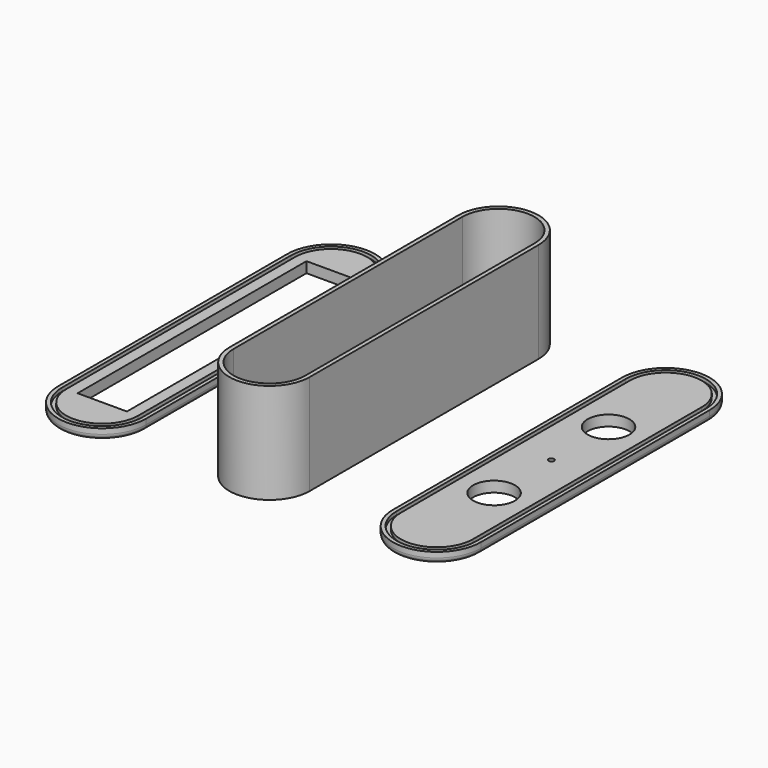
from build123d import *

# Parameters (mm, degrees)
F4_DEPTH  = 12.7
F3_W      = 59
F3_H      = 342.0000019477
F5_DEPTH  = 8.4666666667
F6_D      = 50
F7_D      = 6.5
F9_DEPTH  = 12.7
F10_DEPTH = 8.4666666667
F12_DEPTH = 120
F13_DEPTH = 4.5
F14_D     = 3.5
F15_R     = 6.35
F15_2_R   = 6.35


# Not quite as in the source:
# - a feature names something its author has since deleted; it is built from what else it names


with BuildPart() as f4:
    # F3 (on Top) → F4 (new body)
    with BuildSketch(Plane.XY):
        with BuildLine():
            Line((105, -171), (105, 0))
            Line((105, 0), (105, 171))
            ThreePointArc((105, 171), (52.5, 223.5), (0, 171))
            Line((0, 171), (0, 0))
            Line((0, 0), (0, -171))
            ThreePointArc((0, -171), (52.5, -223.5), (105, -171))
        make_face()
        with BuildLine():
            Line((100.5, 171), (100.5, 0))
            Line((100.5, 0), (100.5, -171))
            ThreePointArc((100.5, -171), (52.5, -219), (4.5, -171))
            Line((4.5, -171), (4.5, 0))
            Line((4.5, 0), (4.5, 171))
            ThreePointArc((4.5, 171), (52.5, 219), (100.5, 171))
        make_face(mode=Mode.SUBTRACT)
    extrude(amount=F4_DEPTH)



with BuildPart() as f4b:
    # F3 (on Top) → F4, piece 2 (new body)
    with BuildSketch(Plane.XY):
        with BuildLine():
            Line((9.5, 171.0000009738), (9.5, 0))
            Line((9.5, 0), (9.5, -171.0000009738))
            ThreePointArc((9.5, -171.0000009738), (52.5, -214), (95.5, -171.0000009738))
            Line((95.5, -171.0000009738), (95.5, 0))
            Line((95.5, 0), (95.5, 171.0000009738))
            ThreePointArc((95.5, 171.0000009738), (52.5, 214), (9.5, 171.0000009738))
        make_face()
        with Locations((52.5, 0)):
            Rectangle(F3_W, F3_H, mode=Mode.SUBTRACT)
        with Locations((52.5, 0)):
            Rectangle(F3_W, F3_H)
    extrude(amount=F4_DEPTH)


with BuildPart() as f4_1:
    add(f4.part)

    add(f4b.part)  # F5 merges F4b
    # F3 (on Top) → F5 (join)
    with BuildSketch(Plane.XY):
        with BuildLine():
            Line((105, -171), (105, 0))
            Line((105, 0), (105, 171))
            ThreePointArc((105, 171), (52.5, 223.5), (0, 171))
            Line((0, 171), (0, 0))
            Line((0, 0), (0, -171))
            ThreePointArc((0, -171), (52.5, -223.5), (105, -171))
        make_face()
        with BuildLine():
            Line((100.5, 171), (100.5, 0))
            Line((100.5, 0), (100.5, -171))
            ThreePointArc((100.5, -171), (52.5, -219), (4.5, -171))
            Line((4.5, -171), (4.5, 0))
            Line((4.5, 0), (4.5, 171))
            ThreePointArc((4.5, 171), (52.5, 219), (100.5, 171))
        make_face(mode=Mode.SUBTRACT)
        with BuildLine():
            Line((100.5, -171), (100.5, 0))
            Line((100.5, 0), (100.5, 171))
            ThreePointArc((100.5, 171), (52.5, 219), (4.5, 171))
            Line((4.5, 171), (4.5, 0))
            Line((4.5, 0), (4.5, -171))
            ThreePointArc((4.5, -171), (52.5, -219), (100.5, -171))
        make_face()
        with BuildLine():
            Line((9.5, -171.0000009738), (9.5, 0))
            Line((9.5, 0), (9.5, 171.0000009738))
            ThreePointArc((9.5, 171.0000009738), (52.5, 214), (95.5, 171.0000009738))
            Line((95.5, 171.0000009738), (95.5, 0))
            Line((95.5, 0), (95.5, -171.0000009738))
            ThreePointArc((95.5, -171.0000009738), (52.5, -214), (9.5, -171.0000009738))
        make_face(mode=Mode.SUBTRACT)
        with BuildLine():
            Line((9.5, 171.0000009738), (9.5, 0))
            Line((9.5, 0), (9.5, -171.0000009738))
            ThreePointArc((9.5, -171.0000009738), (52.5, -214), (95.5, -171.0000009738))
            Line((95.5, -171.0000009738), (95.5, 0))
            Line((95.5, 0), (95.5, 171.0000009738))
            ThreePointArc((95.5, 171.0000009738), (52.5, 214), (9.5, 171.0000009738))
        make_face()
        with Locations((52.5, 0)):
            Rectangle(F3_W, F3_H, mode=Mode.SUBTRACT)
    extrude(amount=F5_DEPTH)

    # F6 (through all)
    with Locations(Plane(origin=(0, 0, 0), x_dir=(1, 0, 0), z_dir=(0, 0, -1))):
        with Locations((52.5, 85.5), (52.5, -85.5)):
            Hole(F6_D / 2)

    # F7 (through all)
    with Locations(Plane(origin=(0, 0, 0), x_dir=(1, 0, 0), z_dir=(0, 0, -1))):
        with Locations((52.5, 0)):
            Hole(F7_D / 2)


with BuildPart() as f4_2:
    # F8: moved
    add(f4_1.part.moved(Location((200, 0, 0))))

    # F15
    f15_edges = [f4_2.edges().sort_by_distance(p)[0] for p in [
        (200, 0, 0),
    ]]
    fillet(f15_edges, radius=F15_R)


with BuildPart() as f9:
    # F3 (on Top) → F9 (new body)
    with BuildSketch(Plane.XY):
        with BuildLine():
            Line((105, -171), (105, 0))
            Line((105, 0), (105, 171))
            ThreePointArc((105, 171), (52.5, 223.5), (0, 171))
            Line((0, 171), (0, 0))
            Line((0, 0), (0, -171))
            ThreePointArc((0, -171), (52.5, -223.5), (105, -171))
        make_face()
        with BuildLine():
            Line((100.5, 171), (100.5, 0))
            Line((100.5, 0), (100.5, -171))
            ThreePointArc((100.5, -171), (52.5, -219), (4.5, -171))
            Line((4.5, -171), (4.5, 0))
            Line((4.5, 0), (4.5, 171))
            ThreePointArc((4.5, 171), (52.5, 219), (100.5, 171))
        make_face(mode=Mode.SUBTRACT)
    extrude(amount=F9_DEPTH)



with BuildPart() as f9b:
    # F3 (on Top) → F9, piece 2 (new body)
    with BuildSketch(Plane.XY):
        with BuildLine():
            Line((9.5, 171.0000009738), (9.5, 0))
            Line((9.5, 0), (9.5, -171.0000009738))
            ThreePointArc((9.5, -171.0000009738), (52.5, -214), (95.5, -171.0000009738))
            Line((95.5, -171.0000009738), (95.5, 0))
            Line((95.5, 0), (95.5, 171.0000009738))
            ThreePointArc((95.5, 171.0000009738), (52.5, 214), (9.5, 171.0000009738))
        make_face()
        with Locations((52.5, 0)):
            Rectangle(F3_W, F3_H, mode=Mode.SUBTRACT)
    extrude(amount=F9_DEPTH)


with BuildPart() as f9_1:
    add(f9.part)

    add(f9b.part)  # F10 merges F9b
    # F3 (on Top) → F10 (join)
    with BuildSketch(Plane.XY):
        with BuildLine():
            Line((100.5, -171), (100.5, 0))
            Line((100.5, 0), (100.5, 171))
            ThreePointArc((100.5, 171), (52.5, 219), (4.5, 171))
            Line((4.5, 171), (4.5, 0))
            Line((4.5, 0), (4.5, -171))
            ThreePointArc((4.5, -171), (52.5, -219), (100.5, -171))
        make_face()
        with BuildLine():
            Line((9.5, -171.0000009738), (9.5, 0))
            Line((9.5, 0), (9.5, 171.0000009738))
            ThreePointArc((9.5, 171.0000009738), (52.5, 214), (95.5, 171.0000009738))
            Line((95.5, 171.0000009738), (95.5, 0))
            Line((95.5, 0), (95.5, -171.0000009738))
            ThreePointArc((95.5, -171.0000009738), (52.5, -214), (9.5, -171.0000009738))
        make_face(mode=Mode.SUBTRACT)
    extrude(amount=F10_DEPTH)


with BuildPart() as f9_2:
    # F11: moved
    add(f9_1.part.moved(Location((-200, 0, 0))))

    # F15#2
    f15_2_edges = [f9_2.edges().sort_by_distance(p)[0] for p in [
        (-95, 0, 0),
    ]]
    fillet(f15_2_edges, radius=F15_2_R)


with BuildPart() as f12:
    # F3 (on Top) → F12 (new body)
    with BuildSketch(Plane.XY):
        with BuildLine():
            Line((100.5, -171), (100.5, 0))
            Line((100.5, 0), (100.5, 171))
            ThreePointArc((100.5, 171), (52.5, 219), (4.5, 171))
            Line((4.5, 171), (4.5, 0))
            Line((4.5, 0), (4.5, -171))
            ThreePointArc((4.5, -171), (52.5, -219), (100.5, -171))
        make_face()
        with BuildLine():
            Line((9.5, -171.0000009738), (9.5, 0))
            Line((9.5, 0), (9.5, 171.0000009738))
            ThreePointArc((9.5, 171.0000009738), (52.5, 214), (95.5, 171.0000009738))
            Line((95.5, 171.0000009738), (95.5, 0))
            Line((95.5, 0), (95.5, -171.0000009738))
            ThreePointArc((95.5, -171.0000009738), (52.5, -214), (9.5, -171.0000009738))
        make_face(mode=Mode.SUBTRACT)
    extrude(amount=F12_DEPTH)


with BuildPart() as f13:
    # F3 (on Top) → F13 (new body)
    with BuildSketch(Plane.XY):
        with BuildLine():
            Line((9.5, 171.0000009738), (9.5, 0))
            Line((9.5, 0), (9.5, -171.0000009738))
            ThreePointArc((9.5, -171.0000009738), (52.5, -214), (95.5, -171.0000009738))
            Line((95.5, -171.0000009738), (95.5, 0))
            Line((95.5, 0), (95.5, 171.0000009738))
            ThreePointArc((95.5, 171.0000009738), (52.5, 214), (9.5, 171.0000009738))
        make_face()
        with Locations((52.5, 0)):
            Rectangle(F3_W, F3_H, mode=Mode.SUBTRACT)
        with Locations((52.5, 0)):
            Rectangle(F3_W, F3_H)
    extrude(amount=F13_DEPTH)

    # F14 (through all)
    with Locations(Plane(origin=(0, 0, 0), x_dir=(1, 0, 0), z_dir=(0, 0, -1))):
        with Locations((16.25, 171.0000009738), (88.75, 171.0000009738), (16.25, -171.0000009738), (88.75, -171.0000009738)):
            Hole(F14_D / 2)


solid = Compound([f4_2.part, f9_2.part, f12.part, f13.part])
